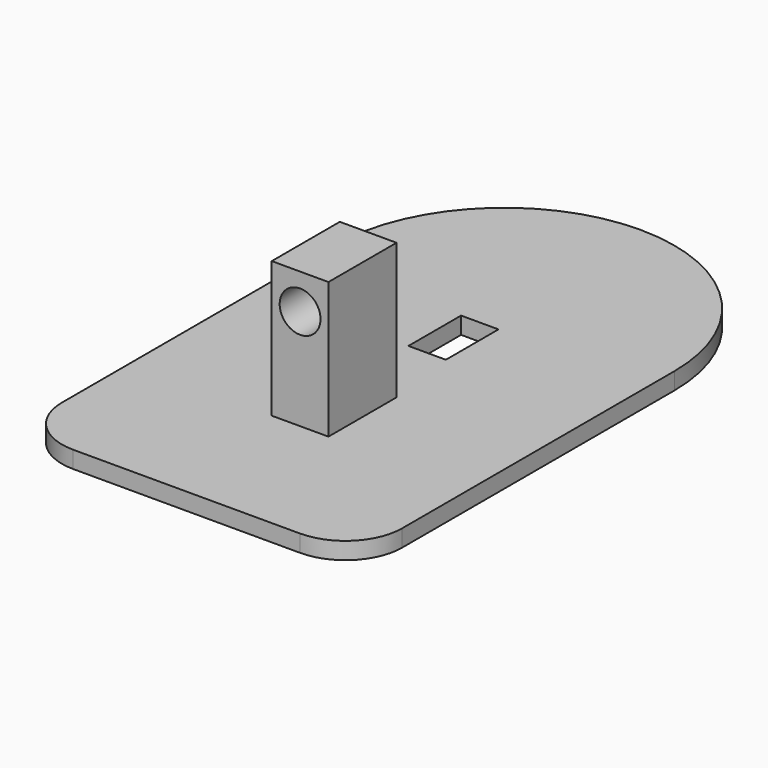
from build123d import *

# Parameters (mm, degrees)
F1_DEPTH = 15
F2_W     = 33
F2_H     = 58
F3_DEPTH = 15.001
F4_W     = 50
F4_H     = 75
F5_DEPTH = 120
F6_R     = 18
F7_DEPTH = 75


# Not quite as in the source:
# - a feature of the source that left no trace in its solid (it failed there, or was rolled back) is left out


with BuildPart() as f1:
    # F0 (on Top) → F1 (new body)
    with BuildSketch(Plane.XY):
        with BuildLine():
            Line((-100, -250), (100, -250))
            ThreePointArc((100, -250), (135.3553390593, -235.3553390593), (150, -200))
            Line((150, -200), (150, 100))
            ThreePointArc((150, 100), (0, 250), (-150, 100))
            Line((-150, 100), (-150, -200))
            ThreePointArc((-150, -200), (-135.3553390593, -235.3553390593), (-100, -250))
        make_face()
    extrude(amount=F1_DEPTH)

    # F2 (on face) → F3 (cut, through all)
    with BuildSketch(Plane.XY.offset(15)):
        with Locations((0, 44)):
            Rectangle(F2_W, F2_H)
    extrude(amount=-F3_DEPTH, mode=Mode.SUBTRACT)

    # F4 (on face) → F5 (join)
    with BuildSketch(Plane.XY.offset(15)):
        with Locations((0, -87.5)):
            Rectangle(F4_W, F4_H)
    extrude(amount=F5_DEPTH)

    # F6 (on face) → F7 (cut, through all)
    with BuildSketch(Plane.XZ.offset(125)):
        with Locations((0, 103.9)):
            Circle(F6_R)
    extrude(amount=-F7_DEPTH, mode=Mode.SUBTRACT)


solid = f1.part
